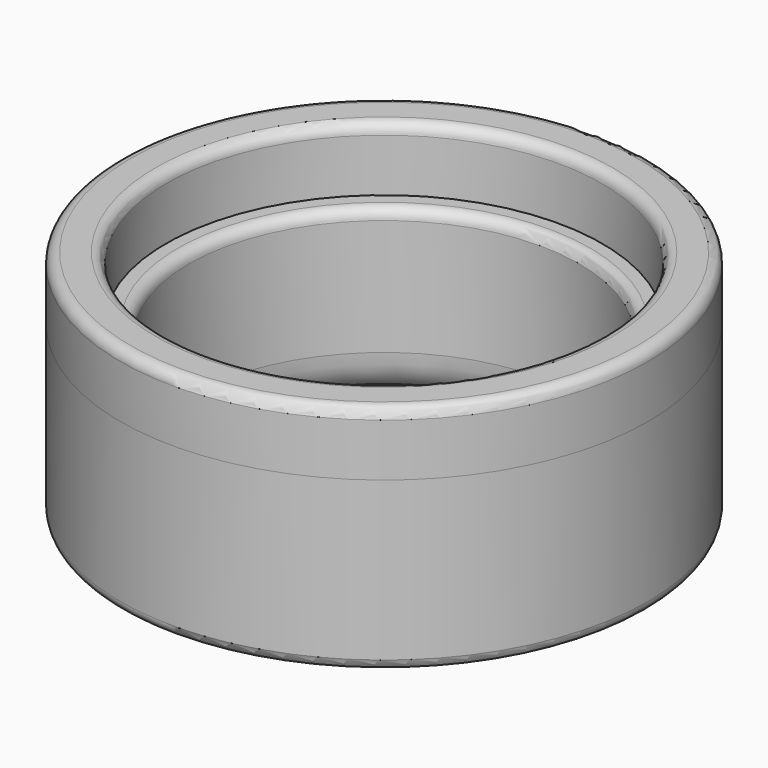
from build123d import *

# Parameters (mm, degrees)
F0_R     = 15.875
F0_R_2   = 13.11275
F0_R_3   = 11.75
F1_DEPTH = 10.16
F2_DEPTH = 3.81
F3_R     = 0.635


# Not quite as in the source:
# - a fillet or chamfer that OpenCascade refuses, or shapes differently, is made with other operations: its cross-section is extruded or revolved along the edge and cut away or added


with BuildPart() as f1:
    # F0 (on Top) → F1 (new body)
    with BuildSketch(Plane.XY):
        Circle(F0_R)
        Circle(F0_R_2, mode=Mode.SUBTRACT)
        Circle(F0_R_2)
        Circle(F0_R_3, mode=Mode.SUBTRACT)
    extrude(amount=-F1_DEPTH)

    # F0 (on Top) → F2 (join)
    with BuildSketch(Plane.XY):
        Circle(F0_R)
        Circle(F0_R_2, mode=Mode.SUBTRACT)
    extrude(amount=F2_DEPTH)

    # F3
    f3_edges = [f1.edges().sort_by_distance(p)[0] for p in [
        (-13.11275, 0, 3.81),
        (-15.875, 0, 3.81),
        (-15.875, 0, -10.16),
        (-11.75, 0, 0),
    ]]
    fillet(f3_edges, radius=F3_R)

    # F4: fillet of radius 2.54 on 1 edges, made by hand

    # F4_s1 → F4_t2 (revolve, cut)
    with BuildSketch(Plane.XZ):
        with BuildLine():
            add(Edge.make_bspline(
                [(14.29, -10.16), (11.75, -10.16), (11.75, -7.62)],
                knots=[0, 0, 0, 1, 1, 1], degree=2, weights=[1, 1, 1]))
            Line((11.75, -7.62), (11.75, -10.16))
            Line((11.75, -10.16), (14.29, -10.16))
        make_face()
    revolve(axis=Axis((0, 0, -10.16), (0, 0, 1)), mode=Mode.SUBTRACT)


solid = f1.part
